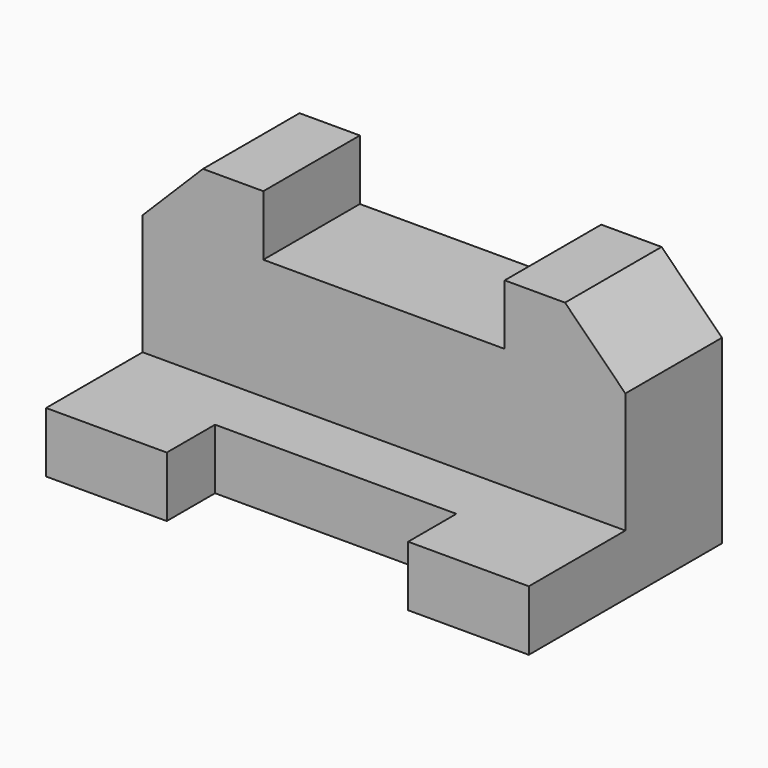
from build123d import *

# Parameters (mm, degrees)
F0_W      = 203.2
F0_H      = 76.2
F1_DEPTH  = 50.8
F2_W      = 203.2
F2_H      = 25.4
F3_DEPTH  = 25.4
F4_W      = 50.8
F4_H      = 25.4
F5_DEPTH  = 25.4
F6_W      = 50.8
F6_H      = 25.4
F7_DEPTH  = 25.4
F8_W      = 25.4
F8_H      = 50.8
F9_DEPTH  = 25.4
F10_SIZE  = 25.39999
F11_W     = 25.4
F11_H     = 50.8
F12_DEPTH = 25.4
F13_W     = 25.4
F13_H     = 50.8
F14_DEPTH = 25.4
F15_SIZE  = 25.39999
F16_W     = 25.4
F16_H     = 50.8
F17_DEPTH = 25.4


# Not quite as in the source:
# - a fillet or chamfer is up to 0.001 mm smaller than in the source, because OpenCascade refuses the exact size


with BuildPart() as f1:
    # F0 (on Front) → F1 (new body)
    with BuildSketch(Plane.XZ):
        with Locations((101.6, 38.1)):
            Rectangle(F0_W, F0_H)
    extrude(amount=F1_DEPTH)

    # F2 (on face) → F3 (join)
    with BuildSketch(Plane.XZ.offset(50.8)):
        with Locations((101.6, 12.7)):
            Rectangle(F2_W, F2_H)
    extrude(amount=F3_DEPTH)

    # F4 (on face) → F5 (join)
    with BuildSketch(Plane.XZ.offset(76.2)):
        with Locations((25.4, 12.7)):
            Rectangle(F4_W, F4_H)
    extrude(amount=F5_DEPTH)

    # F6 (on face) → F7 (join)
    with BuildSketch(Plane.XZ.offset(76.2)):
        with Locations((177.8, 12.7)):
            Rectangle(F6_W, F6_H)
    extrude(amount=F7_DEPTH)

    # F8 (on face) → F9 (join)
    with BuildSketch(Plane.XY.offset(76.2)):
        with Locations((12.7, -25.4)):
            Rectangle(F8_W, F8_H)
    extrude(amount=F9_DEPTH)

    # F10 (size 25.4 in the source; OpenCascade refuses exactly that, so slightly less here)
    f10_edges = [f1.edges().sort_by_distance(p)[0] for p in [
        (0, -25.4, 101.6),
    ]]
    chamfer(f10_edges, length=F10_SIZE)

    # F11 (on face) → F12 (join)
    with BuildSketch(Plane.XY.offset(76.2)):
        with Locations((38.1, -25.4)):
            Rectangle(F11_W, F11_H)
    extrude(amount=F12_DEPTH)

    # F13 (on face) → F14 (join)
    with BuildSketch(Plane.XY.offset(76.2)):
        with Locations((190.5, -25.4)):
            Rectangle(F13_W, F13_H)
    extrude(amount=F14_DEPTH)

    # F15 (size 25.4 in the source; OpenCascade refuses exactly that, so slightly less here)
    f15_edges = [f1.edges().sort_by_distance(p)[0] for p in [
        (203.2, -25.4, 101.6),
    ]]
    chamfer(f15_edges, length=F15_SIZE)

    # F16 (on face) → F17 (join)
    with BuildSketch(Plane.XY.offset(76.2)):
        with Locations((165.1, -25.4)):
            Rectangle(F16_W, F16_H)
    extrude(amount=F17_DEPTH)


solid = f1.part
